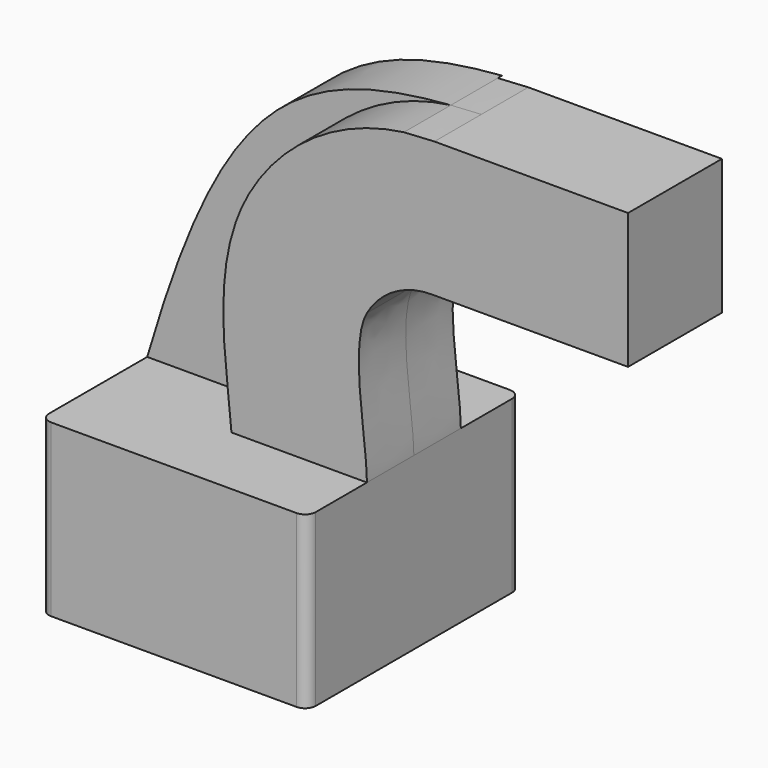
from build123d import *

# Parameters (mm, degrees)
F1_DEPTH = 63.5
F2_DEPTH = 27.94
F3_DEPTH = 30.48
F5_R     = 5.08


# Not quite as in the source:
# - ends of sketch curves that miss each other by under 0.0002 mm in the source are joined
# - the dataset's text gives a spline's control points without its knots; the knots are read off the source's solid
# - the program builds the solid bodies; features that only make, move or delete a surface that nothing else refers to are left out


with BuildPart() as f1:
    # F0 (on Front) → F1 (new body, symmetric)
    with BuildSketch(Plane.XZ):
        Polygon((-63.5, -40.64), (63.5, -40.64), (63.5, 40.64), (-1.0180403389, 40.64), (-63.5, 40.64), align=None)
    extrude(amount=F1_DEPTH, both=True)

    # F0 (on Front) → F2 (join, symmetric)
    with BuildSketch(Plane.XZ):
        with BuildLine():
            Line((-1.0180403389, 40.64), (63.5, 40.64))
            add(Edge.make_bspline(
                [(63.5, 40.64), (63.5, 58.3813676594), (54.7481947164, 96.271286166), (63.5, 111.7037853384)],
                knots=[0, 0, 0, 0, 71.0637853384, 71.0637853384, 71.0637853384, 71.0637853384], degree=3))
            ThreePointArc((63.5, 111.7037853384), (76.4017741745, 124.7558359043), (94.1196627262, 129.54))
            Line((94.1196627262, 129.54), (187.8354665093, 129.54))
            Line((187.8354665093, 129.54), (187.8354665093, 194.0560000929))
            Line((187.8354665093, 194.0560000929), (95.630901588, 194.0560000929))
            add(Edge.make_bspline(
                [(81.099807757, 193.2023550064), (85.7783959014, 193.5638783461), (90.6186920503, 193.8432209612), (95.630901588, 194.0560000929)],
                knots=[219.3887618898, 219.3887618898, 219.3887618898, 219.3887618898, 232.7819441312, 232.7819441312, 232.7819441312, 232.7819441312], degree=3))
            ThreePointArc((81.099807757, 193.2023550064), (38.3986437488, 177.0350565175), (7.3801372504, 143.5294867911))
            add(Edge.make_bspline(
                [(-1.0180403389, 40.64), (-1.0182361302, 40.6459642459), (-1.0193027353, 40.6781499345), (-1.0218795169, 40.7490864596), (-1.0269492868, 40.8703186151), (-1.0338271375, 41.0167364398), (-1.0456053789, 41.2440564869), (-1.0655329065, 41.5857363272), (-1.1094046069, 42.2451333113), (-1.1877043413, 43.2638568381), (-1.3194690546, 44.7534888497), (-1.4869297827, 46.4759329979), (-1.6866993703, 48.4034757344), (-1.91457398, 50.5135844993), (-2.1658549743, 52.7876639481), (-2.5253839158, 56.0180434103), (-3.007640292, 60.3947952335), (-3.5945517267, 66.1119386906), (-4.1416492323, 72.2478132331), (-4.5950562128, 78.784273094), (-4.890089425, 85.7354939883), (-4.9424035401, 93.1558852161), (-4.6298502541, 101.1527940684), (-3.90789741, 108.4437035529), (-2.8882397681, 114.7805587177), (-1.8382156473, 119.8237069223), (-0.4223759869, 125.1947767409), (1.4653498928, 130.9253554886), (3.9592510635, 137.0292943423), (6.134504783, 141.3330003064), (7.3801372504, 143.5294867911)],
                knots=[0.0377648467, 0.0377648467, 0.0377648467, 0.0377648467, 0.0396526905, 0.0473974269, 0.0551421633, 0.0628868996, 0.070631636, 0.0861211087, 0.1016105815, 0.1325895269, 0.1635684724, 0.1945474179, 0.2255263633, 0.2565053088, 0.2874842543, 0.3184631997, 0.3804210907, 0.4423789816, 0.5043368725, 0.5662947635, 0.6282526544, 0.6902105453, 0.7521684363, 0.8141263272, 0.8451052727, 0.8760842181, 0.9070631636, 0.9380421091, 0.9690210545, 1, 1, 1, 1], degree=3))
        make_face()
    extrude(amount=F2_DEPTH, both=True)

    # F0 (on Front) → F3 (join)
    with BuildSketch(Plane.XZ):
        with BuildLine():
            add(Edge.make_bspline(
                [(-63.5, 40.64), (-28.7863279297, 159.3072489949), (4.4615867667, 187.2803749683), (81.099807757, 193.2023550064)],
                knots=[0, 0, 0, 0, 219.3887618898, 219.3887618898, 219.3887618898, 219.3887618898], degree=3))
            Line((-63.5, 40.64), (-1.0180403389, 40.64))
            add(Edge.make_bspline(
                [(-1.0180403389, 40.64), (-1.0182361302, 40.6459642459), (-1.0193027353, 40.6781499345), (-1.0218795169, 40.7490864596), (-1.0269492868, 40.8703186151), (-1.0338271375, 41.0167364398), (-1.0456053789, 41.2440564869), (-1.0655329065, 41.5857363272), (-1.1094046069, 42.2451333113), (-1.1877043413, 43.2638568381), (-1.3194690546, 44.7534888497), (-1.4869297827, 46.4759329979), (-1.6866993703, 48.4034757344), (-1.91457398, 50.5135844993), (-2.1658549743, 52.7876639481), (-2.5253839158, 56.0180434103), (-3.007640292, 60.3947952335), (-3.5945517267, 66.1119386906), (-4.1416492323, 72.2478132331), (-4.5950562128, 78.784273094), (-4.890089425, 85.7354939883), (-4.9424035401, 93.1558852161), (-4.6298502541, 101.1527940684), (-3.90789741, 108.4437035529), (-2.8882397681, 114.7805587177), (-1.8382156473, 119.8237069223), (-0.4223759869, 125.1947767409), (1.4653498928, 130.9253554886), (3.9592510635, 137.0292943423), (6.134504783, 141.3330003064), (7.3801372504, 143.5294867911)],
                knots=[0.0377648467, 0.0377648467, 0.0377648467, 0.0377648467, 0.0396526905, 0.0473974269, 0.0551421633, 0.0628868996, 0.070631636, 0.0861211087, 0.1016105815, 0.1325895269, 0.1635684724, 0.1945474179, 0.2255263633, 0.2565053088, 0.2874842543, 0.3184631997, 0.3804210907, 0.4423789816, 0.5043368725, 0.5662947635, 0.6282526544, 0.6902105453, 0.7521684363, 0.8141263272, 0.8451052727, 0.8760842181, 0.9070631636, 0.9380421091, 0.9690210545, 1, 1, 1, 1], degree=3))
            ThreePointArc((7.3801372504, 143.5294867911), (38.3986437488, 177.0350565175), (81.099807757, 193.2023550064))
        make_face()
    extrude(amount=-F3_DEPTH)

    # F5
    f5_edges = [f1.edges().sort_by_distance(p)[0] for p in [
        (-63.5, -63.5, 0),
        (63.5, -63.5, 0),
        (63.5, 63.5, 0),
        (-63.5, 63.5, 0),
    ]]
    fillet(f5_edges, radius=F5_R)


solid = f1.part
